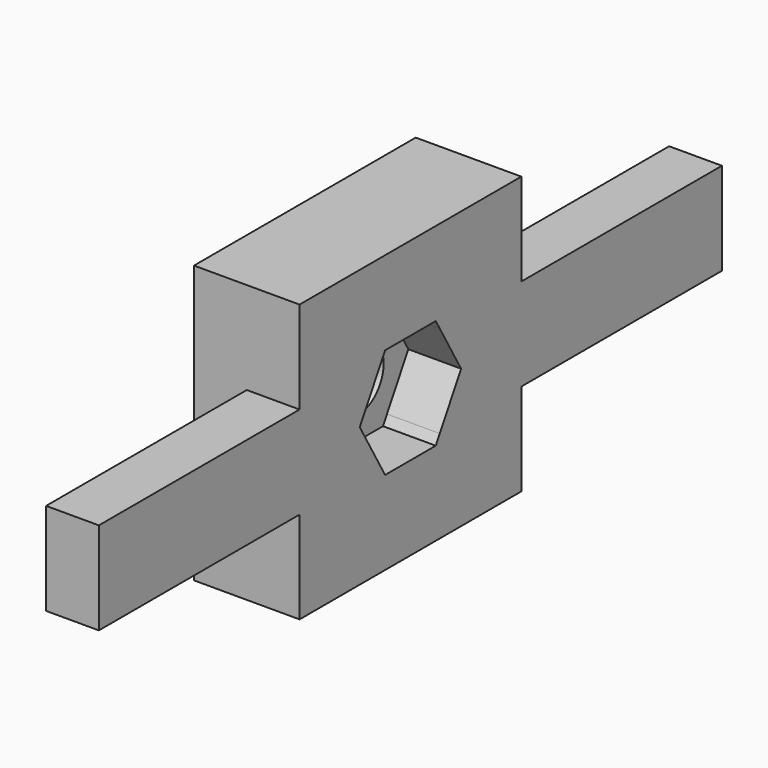
from build123d import *

# Parameters (mm, degrees)
F1_DEPTH = 12.7
F0_R     = 3.9116
F2_DEPTH = 6.35
F3_DEPTH = 6.35


# Not quite as in the source:
# - a length typed as a fraction of an inch, garbled in the dataset ("3 / 203.2 mm" for 3/8 in), is restored


with BuildPart() as f1:
    # F0 (on Right) → F1 (new body)
    with BuildSketch(Plane.YZ):
        Polygon((16.66875, -5.55625), (16.66875, 5.55625), (16.66875, 16.66875), (-16.66875, 16.66875), (-16.66875, 5.55625), (-16.66875, -5.55625), (-16.66875, -5.56895), (-16.66875, -16.66875), (16.66875, -16.66875), (16.66875, -5.56895), align=None)
        Polygon((-4.4120975668, 5.55625), (-3.81, 6.5991135768), (3.81, 6.5991135768), (4.4120975668, 5.55625), (7.62, 0), (4.4120975668, -5.55625), (3.81, -6.5991135768), (-3.81, -6.5991135768), (-4.4120975668, -5.55625), (-7.62, 0), align=None, mode=Mode.SUBTRACT)
        Polygon((-16.66875, -5.55625), (-16.66875, 5.55625), (-46.84395, 5.55625), (-46.84395, -5.56895), (-16.66875, -5.56895), align=None)
        Polygon((46.83125, 5.55625), (16.66875, 5.55625), (16.66875, -5.55625), (16.66875, -5.56895), (46.83125, -5.56895), align=None)
    extrude(amount=F1_DEPTH)

    # F0 (on Right) → F2 (join)
    with BuildSketch(Plane.YZ):
        Polygon((3.81, 6.5991135768), (-3.81, 6.5991135768), (-4.4120975668, 5.55625), (-7.62, 0), (-4.4120975668, -5.55625), (-3.81, -6.5991135768), (3.81, -6.5991135768), (4.4120975668, -5.55625), (7.62, 0), (4.4120975668, 5.55625), align=None)
        Circle(F0_R, mode=Mode.SUBTRACT)
    extrude(amount=F2_DEPTH)

    # F0 (on Right) → F3 (cut)
    with BuildSketch(Plane.YZ):
        Polygon((-16.66875, -5.55625), (-16.66875, 5.55625), (-46.84395, 5.55625), (-46.84395, -5.56895), (-16.66875, -5.56895), align=None)
        Polygon((46.83125, 5.55625), (16.66875, 5.55625), (16.66875, -5.55625), (16.66875, -5.56895), (46.83125, -5.56895), align=None)
    extrude(amount=F3_DEPTH, mode=Mode.SUBTRACT)


solid = f1.part
